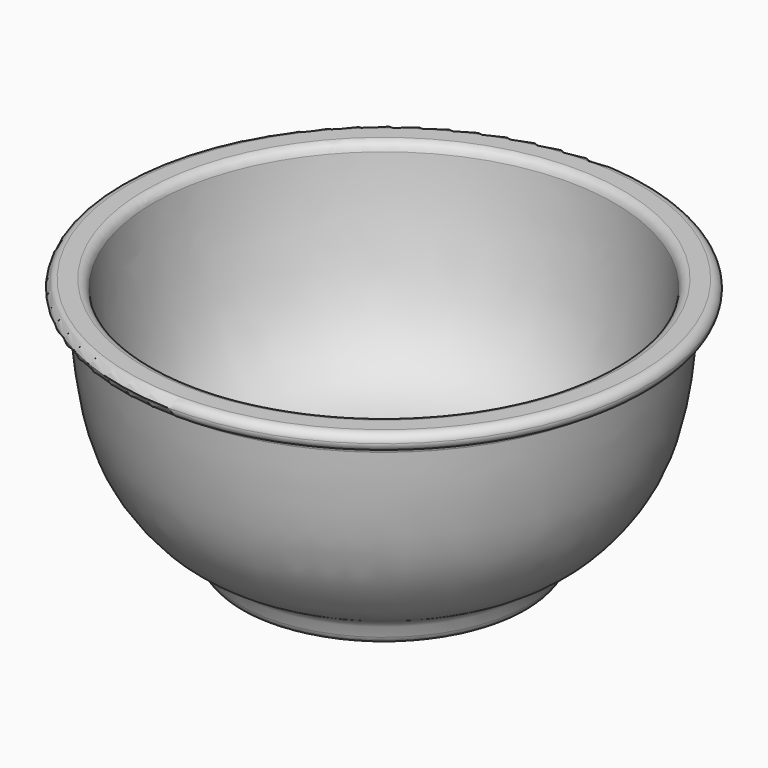
from build123d import *

# Parameters (mm, degrees)
F2_R           = 5.08
F5_D           = 4.4958
F5_CSINK_D     = 9.1186
F5_CSINK_ANGLE = 82


# Not quite as in the source:
# - a fillet or chamfer that OpenCascade refuses, or shapes differently, is made with other operations: its cross-section is extruded or revolved along the edge and cut away or added


with BuildPart() as f1:
    # F0 (on Front) → F1 (revolve)
    with BuildSketch(Plane.XZ):
        with BuildLine():
            Line((35.6394565043, -51.8279158927), (35.6394565043, -39.1279158927))
            Line((35.6394565043, -39.1279158927), (16.5894565043, -39.1279158927))
            Line((16.5894565043, -39.1279158927), (16.5894565043, -26.4279158927))
            add(Edge.make_bspline(
                [(-46.9105434957, 87.8720841073), (-46.4523417325, 82.1133038662), (-45.4505271847, 67.4463326401), (-37.4716489611, 21.6872589154), (-21.5819325296, -8.6134677414), (-2.4548303935, -22.5709949341), (16.5894565043, -26.4279158927)],
                knots=[0, 0, 0, 0, 0.1903258692, 0.4794181484, 0.723894145, 1, 1, 1, 1], degree=3))
            Line((-46.9105434957, 87.8720841073), (-65.9605434957, 87.8720841073))
            Line((-65.9605434957, 87.8720841073), (-65.9605434957, 78.2200841073))
            Line((-65.9605434957, 78.2200841073), (-55.8005434957, 78.2200841073))
            add(Edge.make_bspline(
                [(3.8894565043, -55.0791158927), (3.0613241863, -50.9302523012), (1.7157592211, -40.4137768343), (-15.1746857428, -35.5047598054), (-44.5181155794, -2.9938984023), (-53.5578284027, 42.0725062006), (-55.1225781399, 66.7461177922), (-55.8005434957, 78.2200841073)],
                knots=[0, 0, 0, 0, 0.1345031618, 0.2810038383, 0.5224200823, 0.7767851103, 1, 1, 1, 1], degree=3))
            Line((3.8894565043, -55.0791158927), (16.5894565043, -55.0791158927))
            Line((16.5894565043, -55.0791158927), (16.5894565043, -51.8279158927))
            Line((16.5894565043, -51.8279158927), (35.6394565043, -51.8279158927))
        make_face()
    revolve(axis=Axis((86.4394565043, 0, 3.4914096229), (0, 0, -1)))

    # F2
    f2_edges = [f1.edges().sort_by_distance(p)[0] for p in [
        (228.679457, 0, 78.220084),
        (168.989457, 0, -55.079116),
        (-42.567778, 0, 3.022968),
        (238.839457, 0, 78.220084),
        (219.789457, 0, 87.872084),
    ]]
    fillet(f2_edges, radius=F2_R)

    # F3: fillet of radius 5.08 on 1 edges, made by hand

    # F3_s1 → F3_t2 (revolve, cut)
    with BuildSketch(Plane.XZ):
        with BuildLine():
            ThreePointArc((-65.9605434957, 83.3000841073), (-64.3137749129, 86.5595129387), (-60.9060073152, 87.8720841073))
            Line((-60.9060073152, 87.8720841073), (-65.9605434957, 87.8720841073))
            Line((-65.9605434957, 87.8720841073), (-65.9605434957, 83.3000841073))
        make_face()
    revolve(axis=Axis((86.4394565043, 0, 87.8720841073), (0, 0, -1)), mode=Mode.SUBTRACT)

    # F5 (through all)
    with Locations(Plane(origin=(0, 0, -51.8279158927), x_dir=(1, 0, 0), z_dir=(0, 0, -1))):
        with Locations((116.2203782425, 51.5820695467), (116.2203782425, -51.5820695467), (26.877613028, 0)):
            CounterSinkHole(F5_D / 2, F5_CSINK_D / 2, counter_sink_angle=F5_CSINK_ANGLE)


solid = f1.part
